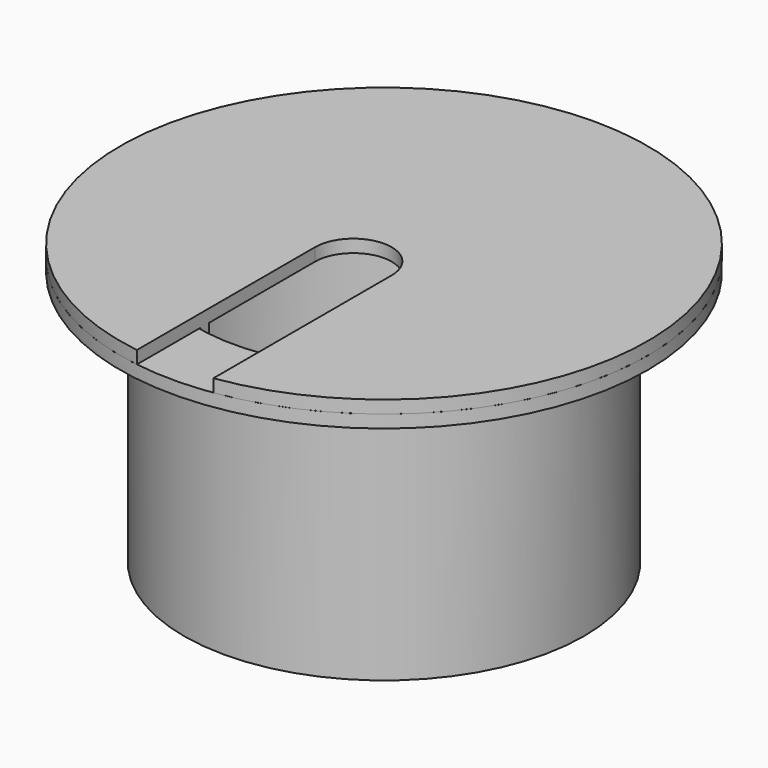
from build123d import *

# Parameters (mm, degrees)
F0_R     = 19.939
F0_R_2   = 18.669
F1_DEPTH = 25.4
F0_R_3   = 26.289
F2_DEPTH = 1.27
F3_R     = 26.289
F4_DEPTH = 1.27
F5_R     = 18.469
F5_R_2   = 17.453
F6_DEPTH = 6.35
F8_DEPTH = 27.941


# Not quite as in the source:
# - a length typed as a fraction of an inch, garbled in the dataset ("3 / 203.2 mm" for 3/8 in), is restored


with BuildPart() as f1:
    # F0 (on Top) → F1 (new body)
    with BuildSketch(Plane.XY):
        Circle(F0_R)
        Circle(F0_R_2, mode=Mode.SUBTRACT)
    extrude(amount=-F1_DEPTH)

    # F0 (on Top) → F2 (join)
    with BuildSketch(Plane.XY):
        Circle(F0_R_3)
        Circle(F0_R, mode=Mode.SUBTRACT)
        Circle(F0_R)
        Circle(F0_R_2, mode=Mode.SUBTRACT)
    extrude(amount=F2_DEPTH)


with BuildPart() as f4:
    # F3 (on face) → F4 (new body)
    with BuildSketch(Plane.XY.offset(1.27)):
        Circle(F3_R)
    extrude(amount=F4_DEPTH)

    # F5 (on face) → F6 (join)
    with BuildSketch(Plane(origin=(0, 0, 1.27), x_dir=(1, 0, 0), z_dir=(0, 0, -1))):
        Circle(F5_R)
        Circle(F5_R_2, mode=Mode.SUBTRACT)
    extrude(amount=F6_DEPTH)

    # F7 (on face) → F8 (cut, through all)
    with BuildSketch(Plane.XY.offset(2.54)):
        with BuildLine():
            Line((3.81, -26.0114478836), (3.81, -3.81))
            ThreePointArc((3.81, -3.81), (0, 0), (-3.81, -3.81))
            Line((-3.81, -3.81), (-3.81, -26.0114478836))
            ThreePointArc((-3.81, -26.0114478836), (0, -26.289), (3.81, -26.0114478836))
        make_face()
    extrude(amount=-F8_DEPTH, mode=Mode.SUBTRACT)


solid = Compound([f1.part, f4.part])
